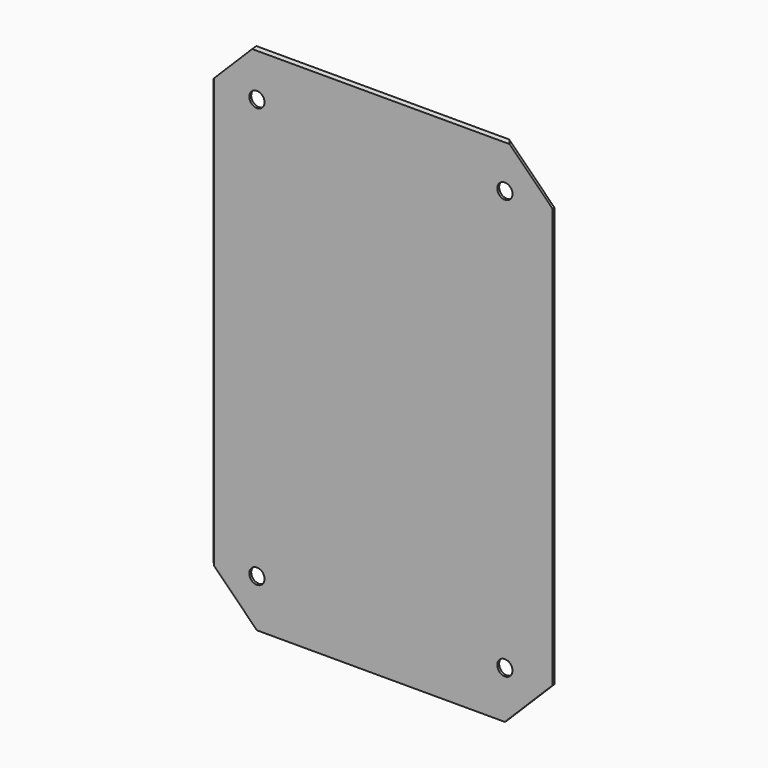
from build123d import *

# Parameters (mm, degrees)
F0_R        = 8
F1_DEPTH    = 2.5
F2_T1_DEPTH = 285.7168298797
F2_T3_DEPTH = 465.7168298797


# Not quite as in the source:
# - a fillet or chamfer that OpenCascade refuses, or shapes differently, is made with other operations: its cross-section is extruded or revolved along the edge and cut away or added


with BuildPart() as f1:
    # F0 (on Front) → F1 (new body)
    with BuildSketch(Plane.XZ):
        Polygon((273.1609285387, 523.1172461575), (13.1609285387, 523.1172461575), (-36.8390714613, 473.1172461575), (-36.8390714613, 33.1172461575), (13.1609285387, -16.8827538425), (273.1609285387, -16.8827538425), (323.1609285387, 33.1172461575), (323.1609285387, 473.1172461575), align=None)
        with Locations((13.1609285387, 33.1172461575)):
            Circle(F0_R, mode=Mode.SUBTRACT)
        with Locations((273.1609285387, 33.1172461575)):
            Circle(F0_R, mode=Mode.SUBTRACT)
        with Locations((13.1609285387, 473.1172461575)):
            Circle(F0_R, mode=Mode.SUBTRACT)
        with Locations((273.1609285387, 473.1172461575)):
            Circle(F0_R, mode=Mode.SUBTRACT)
    extrude(amount=F1_DEPTH)

    # F2: chamfer of 5 on 2 edges, made by hand

    # F2_s2 → F2_t1 (cut)
    with BuildSketch(Plane.YZ.offset(0.3025135989)):
        Polygon((2.5, 523.1172461575), (-2.5, 518.1172461575), (-2.5, 523.1172461575), align=None)
    extrude(amount=F2_T1_DEPTH, mode=Mode.SUBTRACT)

    # F2_s4 → F2_t3 (cut)
    with BuildSketch(Plane.XY.offset(20.2588312177)):
        Polygon((-36.8390714613, 2.5), (-31.8390714613, -2.5), (-36.8390714613, -2.5), align=None)
    extrude(amount=F2_T3_DEPTH, mode=Mode.SUBTRACT)


solid = f1.part
